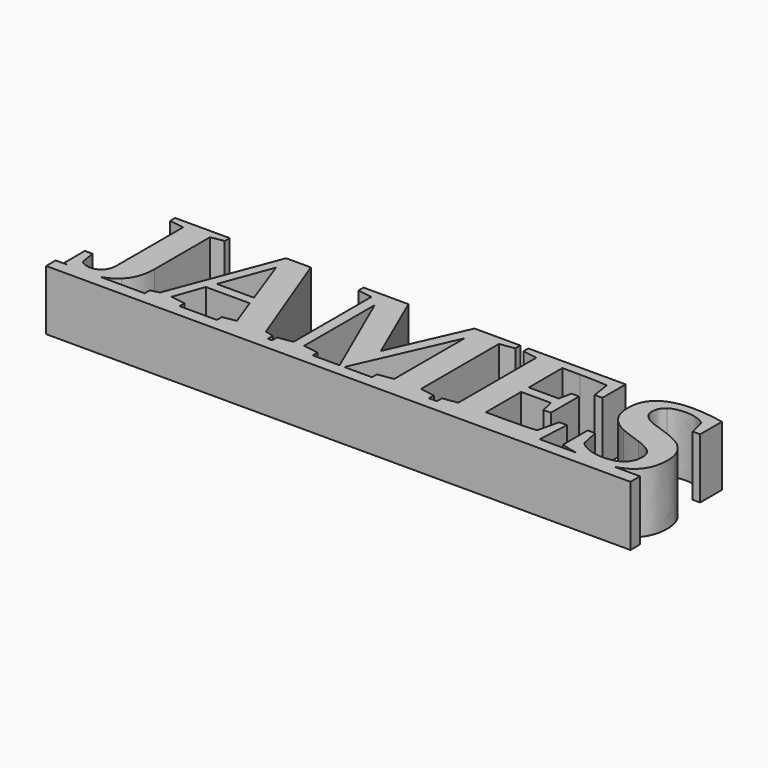
from build123d import *

# Parameters (mm, degrees)
F1_DEPTH = 15


with BuildPart() as f1:
    # F0 (on Top) → F1 (new body)
    with BuildSketch(Plane.XY):
        Polygon((-55.4669993083, -13.3709355081), (-55.4669993083, -14.9245814085), (-46.7788478918, -14.9245814085), (-46.7788478918, -13.3709355081), (-50.4449070777, -12.7917254137), (-47.8282402981, -5.4050931505), (-36.8573196859, -5.4050931505), (-34.1316251238, -12.7917254137), (-37.4365297803, -13.3709355081), (-37.4365297803, -14.9245814085), (-24.7211646484, -14.9245814085), (-24.7211646484, -13.3709355081), (-26.8949060616, -12.7917254137), (-37.0072328868, 13.8655674032), (-43.1809310698, 13.8655674032), (-53.3409575499, -12.7917254137), align=None)
        Polygon((-46.9492038019, -3.0609958272), (-42.2473806823, 9.5657842315), (-37.6682138181, -3.0609958272), align=None, mode=Mode.SUBTRACT)
        with BuildLine():
            Line((-46.7788478918, -14.9245814085), (-55.4669993083, -14.9245814085))
            Line((-55.4669993083, -14.9245814085), (-66.6218982829, -14.9245814085))
            add(Edge.make_bspline(
                [(-66.6218982829, -14.9245814085), (-68.2072820659, -15.353878302), (-70.1653072341, -15.353878302)],
                knots=[0.5859606644, 0.5859606644, 0.5859606644, 1, 1, 1], degree=2))
            add(Edge.make_bspline(
                [(-70.1653072341, -15.353878302), (-71.7598385529, -15.353878302), (-73.3032630987, -15.1698939191)],
                knots=[0, 0, 0, 1, 1, 1], degree=2))
            add(Edge.make_bspline(
                [(-73.3032630987, -15.1698939191), (-74.2052983154, -15.0623665423), (-74.8943654736, -14.9245814085)],
                knots=[0, 0, 0, 0.5844375218, 0.5844375218, 0.5844375218], degree=2))
            Line((-74.8943654736, -14.9245814085), (-77.7018526982, -14.9245814085))
            Line((-77.7018526982, -14.9245814085), (-77.7018526982, -17.9245814085))
            Line((-77.7018526982, -17.9245814085), (68.2590910996, -17.9245814085))
            Line((68.2590910996, -17.9245814085), (68.2590910996, -14.9245814085))
            Line((68.2590910996, -14.9245814085), (61.695634433, -14.9245814085))
            add(Edge.make_bspline(
                [(61.695634433, -14.9245814085), (59.8741275274, -15.353878302), (57.5471114707, -15.353878302)],
                knots=[0.7827650782, 0.7827650782, 0.7827650782, 1, 1, 1], degree=2))
            add(Edge.make_bspline(
                [(57.5471114707, -15.353878302), (55.0939863649, -15.353878302), (52.5488690676, -14.9382098813)],
                knots=[0, 0, 0, 1, 1, 1], degree=2))
            add(Edge.make_bspline(
                [(52.5488690676, -14.9382098813), (52.5073622228, -14.9314309856), (52.4660465805, -14.9245814085)],
                knots=[0, 0, 0, 0.0163084212, 0.0163084212, 0.0163084212], degree=2))
            Line((52.4660465805, -14.9245814085), (43.2099580743, -14.9245814085))
            Line((43.2099580743, -14.9245814085), (17.5066583542, -14.9245814085))
            Line((17.5066583542, -14.9245814085), (15.5032728511, -14.9245814085))
            Line((15.5032728511, -14.9245814085), (1.3024041828, -14.9245814085))
            Line((1.3024041828, -14.9245814085), (-5.6208600048, -14.9245814085))
            Line((-5.6208600048, -14.9245814085), (-6.7929086665, -14.9245814085))
            Line((-6.7929086665, -14.9245814085), (-13.4981172891, -14.9245814085))
            Line((-13.4981172891, -14.9245814085), (-23.6581437692, -14.9245814085))
            Line((-23.6581437692, -14.9245814085), (-24.7211646484, -14.9245814085))
            Line((-24.7211646484, -14.9245814085), (-37.4365297803, -14.9245814085))
            Line((-37.4365297803, -14.9245814085), (-46.7788478918, -14.9245814085))
        make_face()
        with BuildLine():
            add(Edge.make_bspline(
                [(-66.6218982829, -14.9245814085), (-68.2072820659, -15.353878302), (-70.1653072341, -15.353878302)],
                knots=[0.5859606644, 0.5859606644, 0.5859606644, 1, 1, 1], degree=2))
            Line((-66.6218982829, -14.9245814085), (-74.8943654736, -14.9245814085))
            add(Edge.make_bspline(
                [(-73.3032630987, -15.1698939191), (-74.2052983154, -15.0623665423), (-74.8943654736, -14.9245814085)],
                knots=[0, 0, 0, 0.5844375218, 0.5844375218, 0.5844375218], degree=2))
            add(Edge.make_bspline(
                [(-70.1653072341, -15.353878302), (-71.7598385529, -15.353878302), (-73.3032630987, -15.1698939191)],
                knots=[0, 0, 0, 1, 1, 1], degree=2))
        make_face()
        with BuildLine():
            Line((-74.8943654736, -14.9245814085), (-66.6218982829, -14.9245814085))
            add(Edge.make_bspline(
                [(-62.8808885171, -12.8496464231), (-64.3782164513, -14.3170277987), (-66.6218982829, -14.9245814085)],
                knots=[0, 0, 0, 0.5859606644, 0.5859606644, 0.5859606644], degree=2))
            add(Edge.make_bspline(
                [(-60.3255498651, -5.7253622616), (-60.3255498651, -10.3454145443), (-62.8808885171, -12.8496464231)],
                knots=[0, 0, 0, 1, 1, 1], degree=2))
            Line((-60.3255498651, -5.7253622616), (-60.3255498651, 11.5214700798))
            Line((-60.3255498651, 11.5214700798), (-57.0887875727, 12.080237465))
            Line((-57.0887875727, 12.080237465), (-57.0887875727, 13.6338833654))
            Line((-57.0887875727, 13.6338833654), (-70.6968176737, 13.6338833654))
            Line((-70.6968176737, 13.6338833654), (-70.6968176737, 12.080237465))
            Line((-70.6968176737, 12.080237465), (-67.0307584878, 11.5214700798))
            Line((-67.0307584878, 11.5214700798), (-67.0307584878, -9.0438953909))
            add(Edge.make_bspline(
                [(-68.0017871755, -12.0694163548), (-67.0307584878, -11.047280894), (-67.0307584878, -9.0438953909)],
                knots=[0, 0, 0, 1, 1, 1], degree=2))
            add(Edge.make_bspline(
                [(-70.4378766904, -13.0915518155), (-68.9728158632, -13.0915518155), (-68.0017871755, -12.0694163548)],
                knots=[0, 0, 0, 1, 1, 1], degree=2))
            add(Edge.make_bspline(
                [(-72.080107664, -12.8155752411), (-71.3373558958, -13.0915518155), (-70.4378766904, -13.0915518155)],
                knots=[0, 0, 0, 1, 1, 1], degree=2))
            add(Edge.make_bspline(
                [(-73.2317136165, -12.0489736455), (-72.8228594321, -12.5395986667), (-72.080107664, -12.8155752411)],
                knots=[0, 0, 0, 1, 1, 1], degree=2))
            Line((-73.2317136165, -12.0489736455), (-73.8654376021, -8.2398154951))
            Line((-73.8654376021, -8.2398154951), (-75.7666095592, -8.2398154951))
            Line((-75.7666095592, -8.2398154951), (-75.7666095592, -14.7133400799))
            add(Edge.make_bspline(
                [(-74.8943654736, -14.9245814085), (-75.3843245286, -14.8266097186), (-75.7666095592, -14.7133400799)],
                knots=[0.5844375218, 0.5844375218, 0.5844375218, 1, 1, 1], degree=2))
        make_face()
        Polygon((-23.6581437692, -13.3709355081), (-23.6581437692, -14.9245814085), (-13.4981172891, -14.9245814085), (-13.4981172891, -13.3709355081), (-17.3277181488, -12.7917254137), (-17.3277181488, 9.2046297021), (-6.7929086665, -14.9245814085), (-5.6208600048, -14.9245814085), (5.1320050425, 9.2046297021), (5.1320050425, -12.7917254137), (1.3024041828, -13.3709355081), (1.3024041828, -14.9245814085), (15.5032728511, -14.9245814085), (15.5032728511, -13.3709355081), (11.8440279016, -12.7917254137), (11.8440279016, 11.5214700798), (15.5032728511, 12.080237465), (15.5032728511, 13.6338833654), (4.0485414541, 13.6338833654), (-4.278455433, -5.1529664035), (-12.4350964099, 13.6338833654), (-23.6581437692, 13.6338833654), (-23.6581437692, 12.080237465), (-19.9920845832, 11.5214700798), (-19.9920845832, -12.7917254137), align=None)
        with BuildLine():
            add(Edge.make_bspline(
                [(61.695634433, -14.9245814085), (59.8741275274, -15.353878302), (57.5471114707, -15.353878302)],
                knots=[0.7827650782, 0.7827650782, 0.7827650782, 1, 1, 1], degree=2))
            Line((61.695634433, -14.9245814085), (52.4660465805, -14.9245814085))
            add(Edge.make_bspline(
                [(52.5488690676, -14.9382098813), (52.5073622228, -14.9314309856), (52.4660465805, -14.9245814085)],
                knots=[0, 0, 0, 0.0163084212, 0.0163084212, 0.0163084212], degree=2))
            add(Edge.make_bspline(
                [(57.5471114707, -15.353878302), (55.0939863649, -15.353878302), (52.5488690676, -14.9382098813)],
                knots=[0, 0, 0, 1, 1, 1], degree=2))
        make_face()
        with BuildLine():
            Line((52.4660465805, -14.9245814085), (61.695634433, -14.9245814085))
            add(Edge.make_bspline(
                [(68.2590910996, -6.2568727012), (68.2590910996, -13.377691002), (61.695634433, -14.9245814085)],
                knots=[0, 0, 0, 0.7827650782, 0.7827650782, 0.7827650782], degree=2))
            add(Edge.make_bspline(
                [(67.2982837665, -2.1478881489), (68.2590910996, -3.8923326686), (68.2590910996, -6.2568727012)],
                knots=[0, 0, 0, 1, 1, 1], degree=2))
            add(Edge.make_bspline(
                [(64.5180753132, 0.7788263871), (66.3374764333, -0.4034436292), (67.2982837665, -2.1478881489)],
                knots=[0, 0, 0, 1, 1, 1], degree=2))
            add(Edge.make_bspline(
                [(57.8196809269, 3.5624419586), (62.698674193, 1.9610964034), (64.5180753132, 0.7788263871)],
                knots=[0, 0, 0, 1, 1, 1], degree=2))
            add(Edge.make_bspline(
                [(54.1604359774, 5.3579932514), (55.3324846391, 4.3460791452), (57.8196809269, 3.5624419586)],
                knots=[0, 0, 0, 1, 1, 1], degree=2))
            add(Edge.make_bspline(
                [(52.9883873157, 7.7940827662), (52.9883873157, 6.3699073575), (54.1604359774, 5.3579932514)],
                knots=[0, 0, 0, 1, 1, 1], degree=2))
            add(Edge.make_bspline(
                [(54.3921200152, 10.768496957), (52.9883873157, 9.7974682693), (52.9883873157, 7.7940827662)],
                knots=[0, 0, 0, 1, 1, 1], degree=2))
            add(Edge.make_bspline(
                [(58.4193337306, 11.7395256448), (55.7958527146, 11.7395256448), (54.3921200152, 10.768496957)],
                knots=[0, 0, 0, 1, 1, 1], degree=2))
            add(Edge.make_bspline(
                [(63.489125616, 10.1586227988), (61.3153842028, 11.7395256448), (58.4193337306, 11.7395256448)],
                knots=[0, 0, 0, 1, 1, 1], degree=2))
            Line((63.489125616, 10.1586227988), (64.4431187127, 6.2404368658))
            Line((64.4431187127, 6.2404368658), (66.3374764333, 6.2404368658))
            Line((66.3374764333, 6.2404368658), (66.3374764333, 13.0342305617))
            add(Edge.make_bspline(
                [(58.4193337306, 13.9541524764), (61.9968078433, 13.9541524764), (66.3374764333, 13.0342305617)],
                knots=[0, 0, 0, 1, 1, 1], degree=2))
            add(Edge.make_bspline(
                [(50.9134523303, 11.9814310371), (53.4790123369, 13.9541524764), (58.4193337306, 13.9541524764)],
                knots=[0, 0, 0, 1, 1, 1], degree=2))
            add(Edge.make_bspline(
                [(48.3478923238, 6.2404368658), (48.3478923238, 10.0087095979), (50.9134523303, 11.9814310371)],
                knots=[0, 0, 0, 1, 1, 1], degree=2))
            add(Edge.make_bspline(
                [(49.0054661369, 2.6561485167), (48.3478923238, 4.1143951074), (48.3478923238, 6.2404368658)],
                knots=[0, 0, 0, 1, 1, 1], degree=2))
            add(Edge.make_bspline(
                [(50.7703533658, 0.1757664653), (49.66303995, 1.197901926), (49.0054661369, 2.6561485167)],
                knots=[0, 0, 0, 1, 1, 1], degree=2))
            add(Edge.make_bspline(
                [(53.4858265733, -1.6027492365), (51.8776667817, -0.8463689955), (50.7703533658, 0.1757664653)],
                knots=[0, 0, 0, 1, 1, 1], degree=2))
            add(Edge.make_bspline(
                [(58.7600455508, -3.5720635576), (55.0939863649, -2.3591294774), (53.4858265733, -1.6027492365)],
                knots=[0, 0, 0, 1, 1, 1], degree=2))
            add(Edge.make_bspline(
                [(62.4090691458, -5.5107138148), (61.2472418387, -4.4238431082), (58.7600455508, -3.5720635576)],
                knots=[0, 0, 0, 1, 1, 1], degree=2))
            add(Edge.make_bspline(
                [(63.5708964529, -8.171673131), (63.5708964529, -6.5975845214), (62.4090691458, -5.5107138148)],
                knots=[0, 0, 0, 1, 1, 1], degree=2))
            add(Edge.make_bspline(
                [(57.4585263975, -13.200579598), (63.5708964529, -13.200579598), (63.5708964529, -8.171673131)],
                knots=[0, 0, 0, 1, 1, 1], degree=2))
            add(Edge.make_bspline(
                [(53.7141034929, -12.4987132483), (55.5232832584, -13.200579598), (57.4585263975, -13.200579598)],
                knots=[0, 0, 0, 1, 1, 1], degree=2))
            add(Edge.make_bspline(
                [(51.0054445218, -10.7474544922), (51.9049237273, -11.7968468985), (53.7141034929, -12.4987132483)],
                knots=[0, 0, 0, 1, 1, 1], degree=2))
            Line((51.0054445218, -10.7474544922), (50.0514514251, -6.1751018643))
            Line((50.0514514251, -6.1751018643), (48.1775364137, -6.1751018643))
            Line((48.1775364137, -6.1751018643), (48.1775364137, -13.8411178201))
            add(Edge.make_bspline(
                [(52.4660465805, -14.9245814085), (49.9739690811, -14.5114285169), (48.1775364137, -13.8411178201)],
                knots=[0.0163084212, 0.0163084212, 0.0163084212, 1, 1, 1], degree=2))
        make_face()
        with BuildLine():
            Line((17.5066583542, -14.9245814085), (43.2099580743, -14.9245814085))
            Line((43.2099580743, -14.9245814085), (43.6188122587, -6.9587390509))
            Line((43.6188122587, -6.9587390509), (41.6767548832, -6.9587390509))
            Line((41.6767548832, -6.9587390509), (40.4638208031, -12.2397722649))
            add(Edge.make_bspline(
                [(33.2679871593, -12.5804840851), (38.7602617018, -12.5804840851), (40.4638208031, -12.2397722649)],
                knots=[0, 0, 0, 1, 1, 1], degree=2))
            Line((33.2679871593, -12.5804840851), (27.8779261628, -12.5804840851))
            Line((27.8779261628, -12.5804840851), (27.8779261628, -1.5754922909))
            Line((27.8779261628, -1.5754922909), (35.3531434992, -1.5754922909))
            Line((35.3531434992, -1.5754922909), (36.0141244305, -4.8122545833))
            Line((36.0141244305, -4.8122545833), (37.9084821512, -4.8122545833))
            Line((37.9084821512, -4.8122545833), (37.9084821512, 3.9644819065))
            Line((37.9084821512, 3.9644819065), (36.0141244305, 3.9644819065))
            Line((36.0141244305, 3.9644819065), (35.3531434992, 0.8094904509))
            Line((35.3531434992, 0.8094904509), (27.8779261628, 0.8094904509))
            Line((27.8779261628, 0.8094904509), (27.8779261628, 11.289786042))
            Line((27.8779261628, 11.289786042), (32.3071798261, 11.289786042))
            add(Edge.make_bspline(
                [(39.2100013045, 10.9899596402), (36.8250185627, 11.289786042), (32.3071798261, 11.289786042)],
                knots=[0, 0, 0, 1, 1, 1], degree=2))
            Line((39.2100013045, 10.9899596402), (39.8914249451, 6.3699073575))
            Line((39.8914249451, 6.3699073575), (41.8266680841, 6.3699073575))
            Line((41.8266680841, 6.3699073575), (41.8266680841, 13.6338833654))
            Line((41.8266680841, 13.6338833654), (17.5066583542, 13.6338833654))
            Line((17.5066583542, 13.6338833654), (17.5066583542, 12.080237465))
            Line((17.5066583542, 12.080237465), (21.1727175402, 11.5214700798))
            Line((21.1727175402, 11.5214700798), (21.1727175402, -12.7917254137))
            Line((21.1727175402, -12.7917254137), (17.5066583542, -13.3709355081))
            Line((17.5066583542, -13.3709355081), (17.5066583542, -14.9245814085))
        make_face()
    extrude(amount=F1_DEPTH)


solid = f1.part
